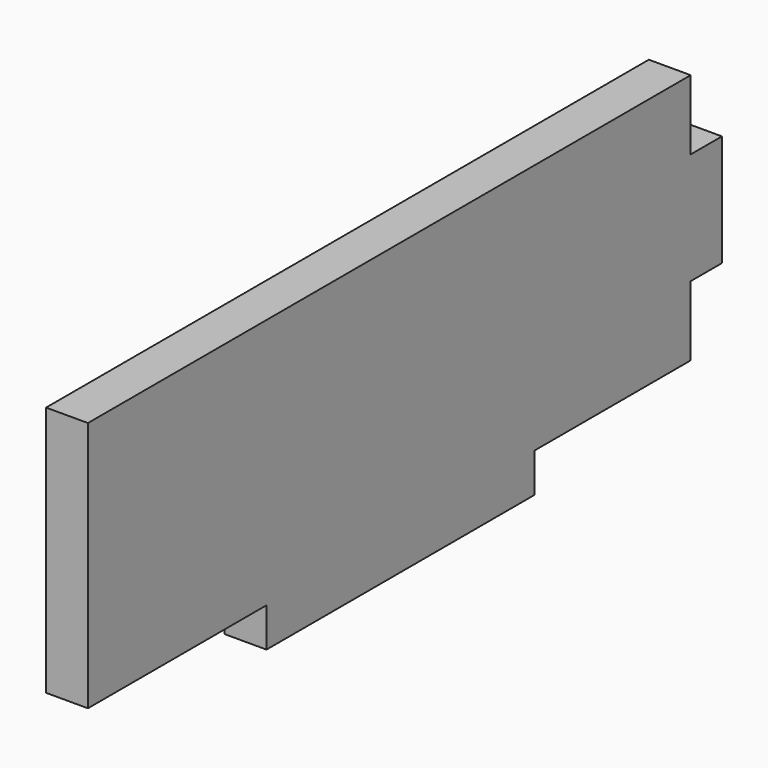
from build123d import *

# Parameters (mm, degrees)
F0_W     = 152.4
F0_H     = 17.78
F0_W_2   = 17.78
F0_H_2   = 50.8
F1_DEPTH = 19.05


# Not quite as in the source:
# - a feature names something its author has since deleted; it is built from what else it names


with BuildPart() as f1:
    # F0 (on Right) → F1 (new body)
    with BuildSketch(Plane.YZ):
        Polygon((171.45, 0), (-171.45, 0), (-171.45, -114.3), (-69.85, -114.3), (82.55, -114.3), (171.45, -114.3), (171.45, -82.55), (171.45, -31.75), align=None)
        with Locations((6.35, -123.19)):
            Rectangle(F0_W, F0_H)
        with Locations((180.34, -57.15)):
            Rectangle(F0_W_2, F0_H_2)
    extrude(amount=F1_DEPTH)


solid = f1.part
